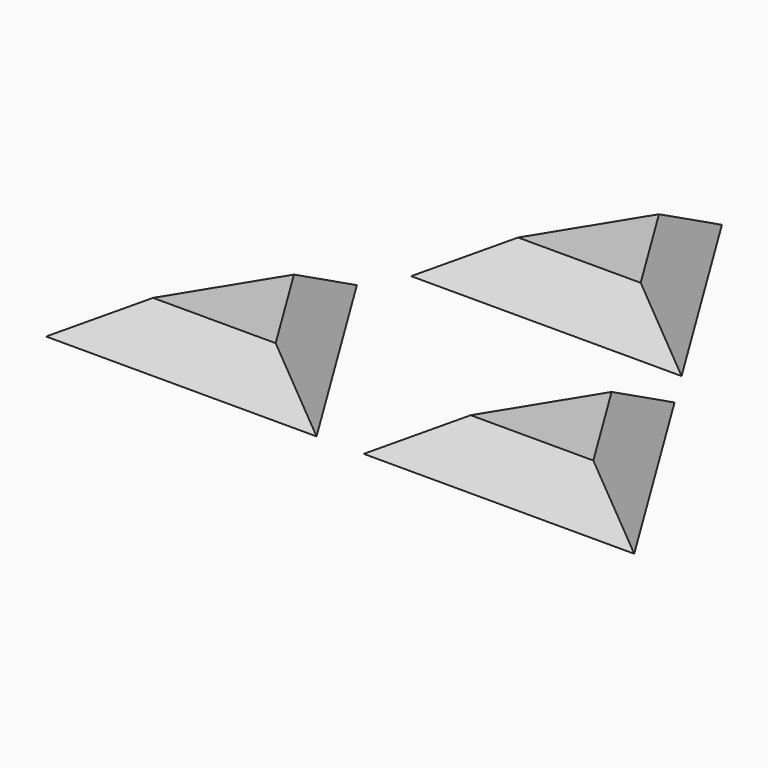
from build123d import *

# Parameters (mm, degrees)
F1_DEPTH      = 5.776533857
F2_T1_DEPTH   = 83.6424487366
F2_T3_DEPTH   = 81.5562575155
F2_T5_DEPTH   = 81.5562575155
F2_2_T1_DEPTH = 83.6424487366
F2_2_T3_DEPTH = 81.5562575155
F2_2_T5_DEPTH = 81.5562575155
F2_3_T1_DEPTH = 81.5562575155
F2_3_T3_DEPTH = 83.6424487366
F2_3_T5_DEPTH = 81.5562575155


# Not quite as in the source:
# - a fillet or chamfer that OpenCascade refuses, or shapes differently, is made with other operations: its cross-section is extruded or revolved along the edge and cut away or added


with BuildPart() as f1:
    # F0 (on Top) → F1 (new body)
    with BuildSketch(Plane.XY):
        Polygon((21.688936314, 24.8060692102), (-0.536063686, -11.25972718), (43.913936314, -11.25972718), align=None)
    extrude(amount=F1_DEPTH)

    # F2: chamfer of 7.62 on 3 edges, made by hand

    # F2_s2 → F2_t1 (cut)
    with BuildSketch(Plane.YZ.offset(-20.1322880543)):
        Polygon((-11.25972718, -1.843466143), (-3.63972718, 5.776533857), (-11.25972718, 5.776533857), align=None)
    extrude(amount=F2_T1_DEPTH, mode=Mode.SUBTRACT)

    # F2_s4 → F2_t3 (cut)
    with BuildSketch(Plane(origin=(27.3959125979, -44.4569361385, 0), x_dir=(0, 0, 1), z_dir=(-0.5246223284, 0.8513350766, 0))):
        Polygon((-1.843466143, 31.478370044), (5.776533857, 23.858370044), (5.776533857, 31.478370044), align=None)
    extrude(amount=F2_T3_DEPTH, mode=Mode.SUBTRACT)

    # F2_s6 → F2_t5 (cut)
    with BuildSketch(Plane(origin=(27.3291517213, 44.3485993924, 0), x_dir=(0, 0, 1), z_dir=(-0.5246223284, -0.8513350766, 0))):
        Polygon((-1.843466143, -5.4507344708), (5.776533857, -13.0707344708), (5.776533857, -5.4507344708), align=None)
    extrude(amount=F2_T5_DEPTH, mode=Mode.SUBTRACT)


with BuildPart() as f1b:
    # F0 (on Top) → F1, piece 2 (new body)
    with BuildSketch(Plane.XY):
        Polygon((-22.761063686, 24.8060692102), (-44.986063686, -11.25972718), (-0.536063686, -11.25972718), align=None)
    extrude(amount=F1_DEPTH)

    # F2#2: chamfer of 7.62 on 3 edges, made by hand

    # F2_2_s2 → F2_2_t1 (cut)
    with BuildSketch(Plane.YZ.offset(-64.5822880543)):
        Polygon((-11.25972718, -1.843466143), (-3.63972718, 5.776533857), (-11.25972718, 5.776533857), align=None)
    extrude(amount=F2_2_T1_DEPTH, mode=Mode.SUBTRACT)

    # F2_2_s4 → F2_2_t3 (cut)
    with BuildSketch(Plane(origin=(15.1620018871, -24.6042597493, 0), x_dir=(0, 0, 1), z_dir=(-0.5246223284, 0.8513350766, 0))):
        Polygon((-1.843466143, -6.3634741091), (5.776533857, -13.9834741091), (5.776533857, -6.3634741091), align=None)
    extrude(amount=F2_2_T3_DEPTH, mode=Mode.SUBTRACT)

    # F2_2_s6 → F2_2_t5 (cut)
    with BuildSketch(Plane(origin=(15.0952410105, 24.4959230032, 0), x_dir=(0, 0, 1), z_dir=(-0.5246223284, -0.8513350766, 0))):
        Polygon((-1.843466143, 32.3911096823), (5.776533857, 24.7711096823), (5.776533857, 32.3911096823), align=None)
    extrude(amount=F2_2_T5_DEPTH, mode=Mode.SUBTRACT)


with BuildPart() as f1c:
    # F0 (on Top) → F1, piece 3 (new body)
    with BuildSketch(Plane.XY):
        Polygon((-0.536063686, 60.8718656003), (-22.761063686, 24.8060692102), (21.688936314, 24.8060692102), align=None)
    extrude(amount=F1_DEPTH)

    # F2#3: chamfer of 7.62 on 3 edges, made by hand

    # F2_3_s2 → F2_3_t1 (cut)
    with BuildSketch(Plane(origin=(37.3202410105, 60.5617193934, 0), x_dir=(0, 0, 1), z_dir=(-0.5246223284, -0.8513350766, 0))):
        Polygon((-1.843466143, 32.3911096823), (5.776533857, 24.7711096823), (5.776533857, 32.3911096823), align=None)
    extrude(amount=F2_3_T1_DEPTH, mode=Mode.SUBTRACT)

    # F2_3_s4 → F2_3_t3 (cut)
    with BuildSketch(Plane.YZ.offset(-42.3572880543)):
        Polygon((24.8060692102, -1.843466143), (32.4260692102, 5.776533857), (24.8060692102, 5.776533857), align=None)
    extrude(amount=F2_3_T3_DEPTH, mode=Mode.SUBTRACT)

    # F2_3_s6 → F2_3_t5 (cut)
    with BuildSketch(Plane(origin=(5.1709125979, -8.3911397483, 0), x_dir=(0, 0, 1), z_dir=(-0.5246223284, 0.8513350766, 0))):
        Polygon((-1.843466143, 31.478370044), (5.776533857, 23.858370044), (5.776533857, 31.478370044), align=None)
    extrude(amount=F2_3_T5_DEPTH, mode=Mode.SUBTRACT)


solid = Compound([f1.part, f1b.part, f1c.part])
